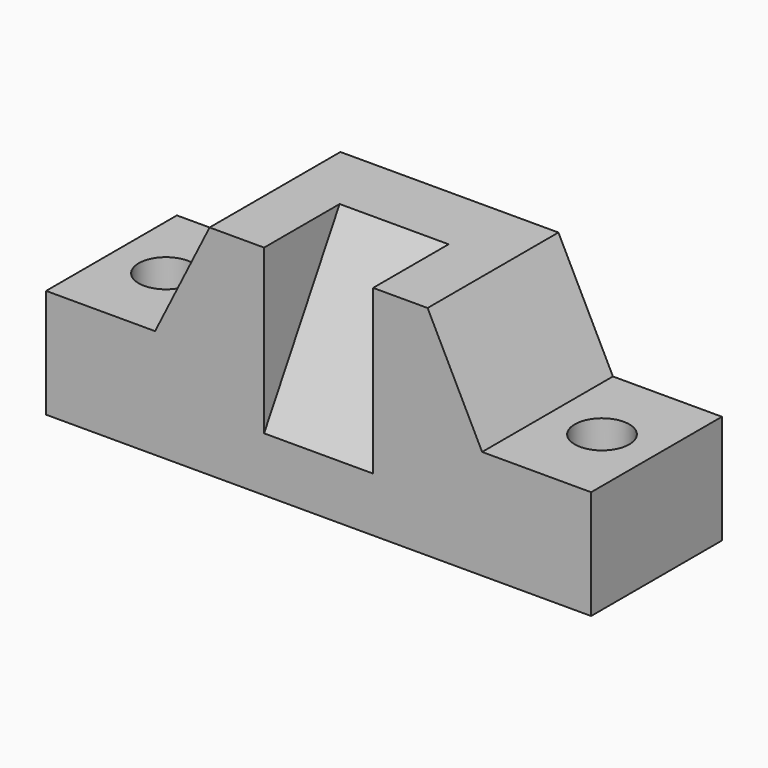
from build123d import *

# Parameters (mm, degrees)
F1_DEPTH = 38.1
F3_D     = 12.7
F5_START = -50.8
F5_DEPTH = 25.4


# Not quite as in the source:
# - a length typed as a fraction of an inch, garbled in the dataset ("3 / 203.2 mm" for 3/8 in), is restored


with BuildPart() as f1:
    # F0 (on Front) → F1 (new body)
    with BuildSketch(Plane.XZ):
        Polygon((-63.5, 0), (63.5, 0), (63.5, 25.4), (38.1, 25.4), (25.4, 50.8), (-25.4, 50.8), (-38.1, 25.4), (-63.5, 25.4), align=None)
    extrude(amount=-F1_DEPTH)

    # F3 (through all)
    with Locations(Plane.XY.offset(25.4)):
        with Locations((-50.8, 19.05), (50.8, 19.05)):
            Hole(F3_D / 2)

    # F4 (on face) → F5 (cut)
    with BuildSketch(Plane.YZ.offset(63.5).offset(F5_START)):
        Polygon((0, 25.4), (7.3323484187, 25.4), (21.9970452561, 50.8), (0, 50.8), align=None)
        Polygon((0, 25.4), (0, 12.7), (7.3323484187, 25.4), align=None)
    extrude(amount=-F5_DEPTH, mode=Mode.SUBTRACT)


solid = f1.part
